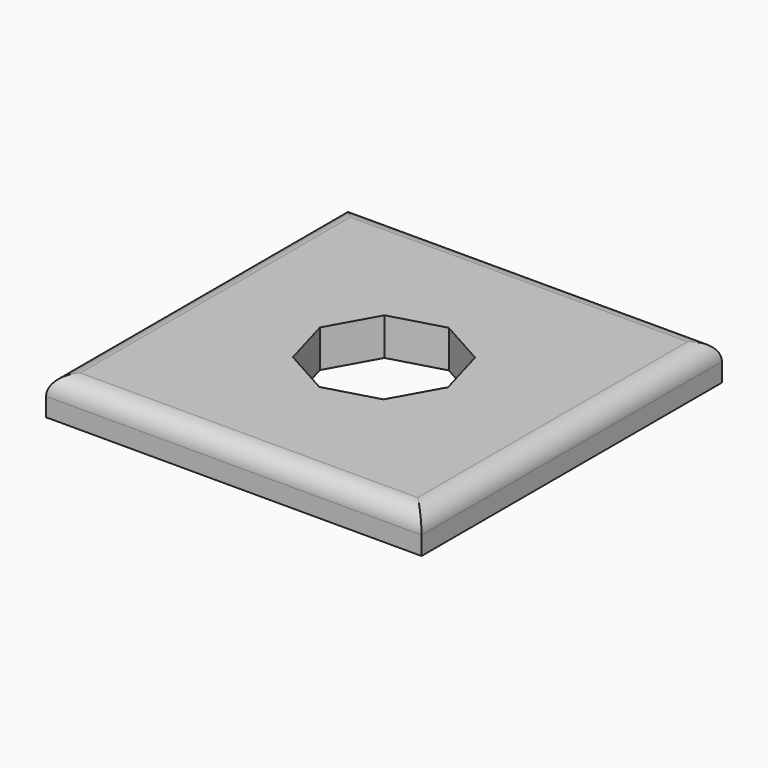
from build123d import *

# Parameters (mm, degrees)
F0_W     = 100
F0_H     = 100
F2_DEPTH = 10
F3_R     = 5.08
F4_DEPTH = 61.976


# Not quite as in the source:
# - a feature of the source that left no trace in its solid (it failed there, or was rolled back) is left out


with BuildPart() as f2:
    # F0 (on Top) → F2 (new body)
    with BuildSketch(Plane.XY):
        Rectangle(F0_W, F0_H)
    extrude(amount=F2_DEPTH)

    # F3
    f3_edges = [f2.edges().sort_by_distance(p)[0] for p in [
        (0, 50, 10),
        (-50, 0, 10),
        (0, -50, 10),
        (50, 0, 10),
    ]]
    fillet(f3_edges, radius=F3_R)

    # F1 (on face) → F4 (cut)
    with BuildSketch(Plane.XY):
        Polygon((-11.7515370065, 14.8558261646), (-18.8142469277, 2.1950639145), (-14.8558261646, -11.7515370065), (-2.1950639145, -18.8142469277), (11.7515370065, -14.8558261646), (18.8142469277, -2.1950639145), (14.8558261646, 11.7515370065), (2.1950639145, 18.8142469277), align=None)
    extrude(amount=F4_DEPTH, mode=Mode.SUBTRACT)


solid = f2.part
